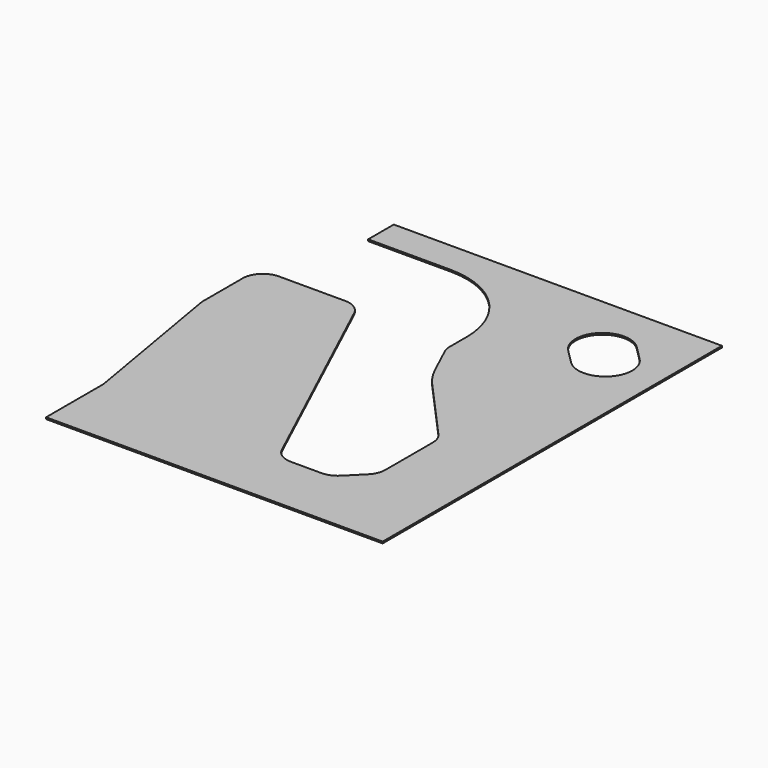
from build123d import *

# Parameters (mm, degrees)
F1_DEPTH = 12.7


# Not quite as in the source:
# - ends of sketch curves that miss each other by under 0.0002 mm in the source are joined


with BuildPart() as f1:
    # F0 (on Top) → F1 (new body)
    with BuildSketch(Plane.XY):
        with BuildLine():
            Line((-4869.3159662, 1221.4318472), (-7345.8159662, 1221.4318472))
            Line((-7345.8159662, 1221.4318472), (-7345.8159662, 980.1318472))
            Line((-7345.8159662, 980.1318472), (-6723.5159662, 980.1318472))
            ThreePointArc((-6723.5159662, 980.1318472), (-6292.4636723887, 801.5841410113), (-6113.9159662, 370.5318472))
            Line((-6113.9159662, 370.5318472), (-6113.9159662, 209.4173104))
            ThreePointArc((-6113.9159662, 209.4173104), (-6110.325234886, 176.5302072569), (-6099.7222450301, 145.1928252566))
            Line((-6099.7222450301, 145.1928252566), (-5997.202636, -75.4216932))
            ThreePointArc((-5997.202636, -75.4216932), (-5953.1314034471, -154.3535570901), (-5897.8716226826, -225.8998318064))
            Line((-5897.8716226826, -225.8998318064), (-5467.1424566, -705.3907914))
            ThreePointArc((-5467.1424566, -705.3907914), (-5438.2066479658, -752.7020855956), (-5428.1159662, -807.2348092))
            Line((-5428.1159662, -807.2348092), (-5428.1159662, -1254.384588))
            ThreePointArc((-5428.1159662, -1254.384588), (-5439.7167254453, -1312.7055430924), (-5472.7528927472, -1362.1476614528))
            Line((-5472.7528927472, -1362.1476614528), (-5587.736475, -1477.1312088))
            ThreePointArc((-5587.736475, -1477.1312088), (-5637.1785759076, -1510.1673935547), (-5695.499531, -1521.7681528))
            Line((-5695.499531, -1521.7681528), (-5928.068281, -1521.7681528))
            ThreePointArc((-5928.068281, -1521.7681528), (-6010.0376303452, -1497.8468894373), (-6066.2745598301, -1433.5926379434))
            Line((-6066.2745598301, -1433.5926379434), (-6822.3645112, 193.4563314))
            ThreePointArc((-6822.3645112, 193.4563314), (-6878.6014386548, 257.7105838373), (-6960.570788, 281.6318472))
            Line((-6960.570788, 281.6318472), (-7460.1159662, 281.6318472))
            ThreePointArc((-7460.1159662, 281.6318472), (-7567.8790396528, 236.9949206528), (-7612.5159662, 129.2318472))
            Line((-7612.5159662, 129.2318472), (-7612.5159662, -242.3205212))
            ThreePointArc((-7612.5159662, -242.3205212), (-7611.9634211451, -255.2862616993), (-7610.3097926213, -268.1579844059))
            Line((-7610.3097926213, -268.1579844059), (-7411.5221594, -1423.7158978))
            ThreePointArc((-7411.5221594, -1423.7158978), (-7409.8685114381, -1436.5876193554), (-7409.3159662, -1449.553362))
            Line((-7409.3159662, -1449.553362), (-7409.3159662, -1978.9681528))
            Line((-7409.3159662, -1978.9681528), (-4869.3159662, -1978.9681528))
            Line((-4869.3159662, -1978.9681528), (-4869.3159662, 1221.4318472))
        make_face()
        with BuildLine():
            ThreePointArc((-5538.4318936371, 607.8479651629), (-5538.4318809371, 895.2161483371), (-5251.0636977629, 895.2161610371))
            Line((-5251.0636977629, 895.2161610371), (-5143.3005338, 787.4531622))
            ThreePointArc((-5143.3005338, 787.4531622), (-5143.3005274629, 500.0849472629), (-5430.6687360371, 500.0849599629))
            Line((-5430.6687360371, 500.0849599629), (-5538.4318936371, 607.8479651629))
        make_face(mode=Mode.SUBTRACT)
    extrude(amount=F1_DEPTH)


solid = f1.part
